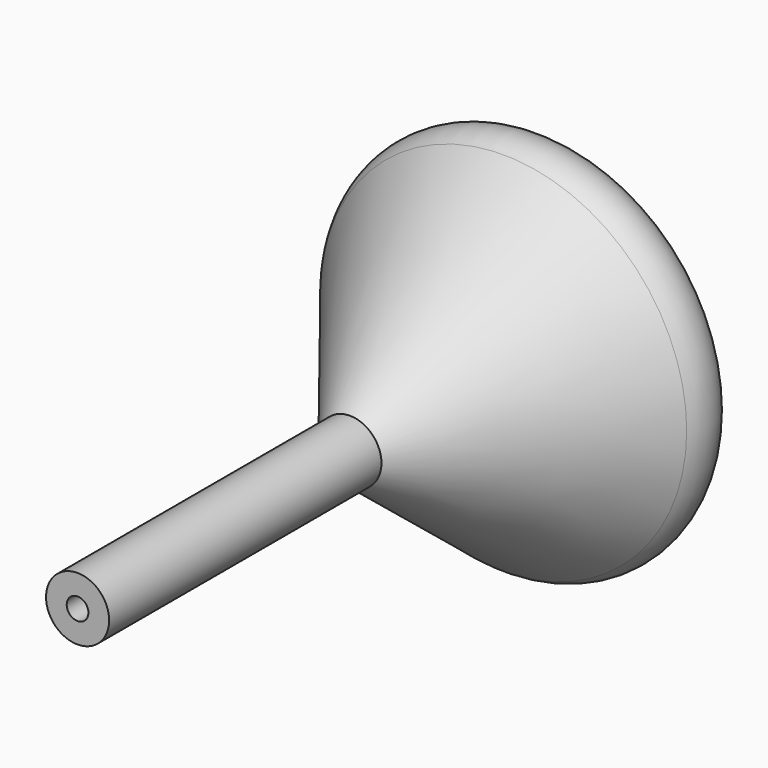
from build123d import *

# Parameters (mm, degrees)
F2_R     = 1.5533685179
F3_DEPTH = 50.8


# Not quite as in the source:
# - a fillet or chamfer that OpenCascade refuses, or shapes differently, is made with other operations: its cross-section is extruded or revolved along the edge and cut away or added


with BuildPart() as f1:
    # F0 (on Top) → F1 (revolve)
    with BuildSketch(Plane.XY):
        Polygon((25.7452992698, 34.3298881523), (0, 0), (0, -48.7618558109), (4.5166942291, -48.7618558109), (4.5166942291, 0), (29.4045954943, 31.4324982464), align=None)
    revolve(axis=Axis((0, -24.3809279054, 0), (0, -1, 0)))

    # F2 (on face) → F3 (cut)
    with BuildSketch(Plane.XZ.offset(48.7618558109)):
        Circle(F2_R)
    extrude(amount=-F3_DEPTH, mode=Mode.SUBTRACT)

    # F4: fillet of radius 5.08 on 1 edges, made by hand

    # F4_s1 → F4_t2 (revolve, cut)
    with BuildSketch(Plane.XY):
        with BuildLine():
            ThreePointArc((25.7452992698, 34.3298881523), (27.3445295723, 30.9972333724), (26.261540234, 27.4629357709))
            Line((26.261540234, 27.4629357709), (26.3411945536, 27.3998663697))
            Line((26.3411945536, 27.3998663697), (29.4842498139, 31.3694288452))
            Line((29.4842498139, 31.3694288452), (29.4676648955, 31.5121525661))
            ThreePointArc((29.4676648955, 31.5121525661), (27.6380167832, 32.960847519), (25.8146287701, 34.4041577987))
            Line((25.8146287701, 34.4041577987), (25.7452992698, 34.3298881523))
        make_face()
    revolve(axis=Axis((0, 31.4324982464, 0), (0, -1, 0)), mode=Mode.SUBTRACT)


solid = f1.part
